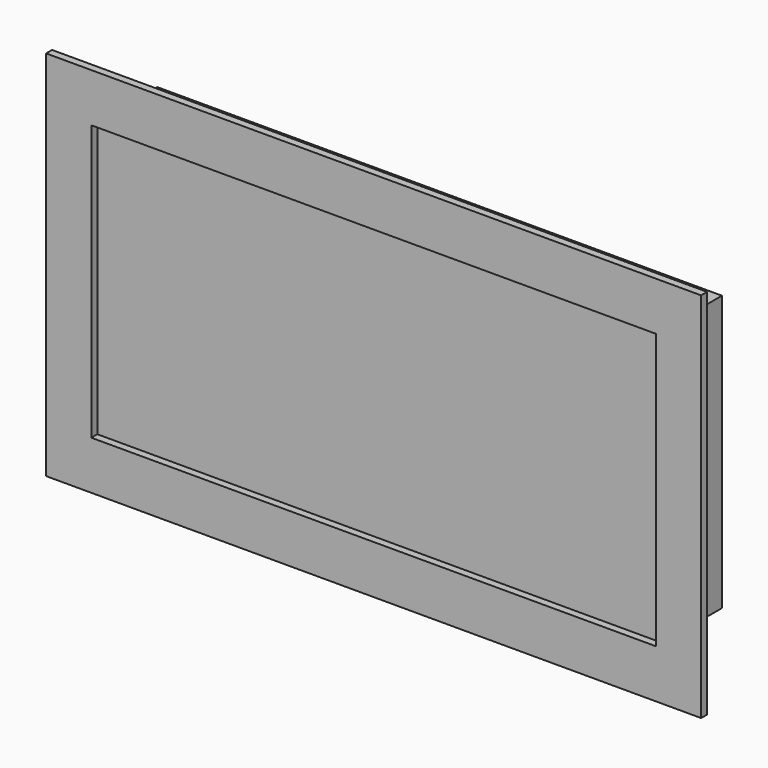
from build123d import *

# Parameters (mm, degrees)
F3_W     = 191.1528706551
F3_H     = 93.1293070316
F0_DEPTH = 25.4
F3_W_2   = 221.7658758163
F3_H_2   = 125.9914338589
F1_DEPTH = 2.54


# Not quite as in the source:
# - a feature of the source that left no trace in its solid (it failed there, or was rolled back) is left out


with BuildPart() as f0:
    # F3 (on Front) → F0 (new body)
    with BuildSketch(Plane.XZ):
        Rectangle(F3_W, F3_H)
    extrude(amount=-F0_DEPTH)


with BuildPart() as f1:
    # F3 (on Front) → F1 (new body)
    with BuildSketch(Plane.XZ):
        Rectangle(F3_W_2, F3_H_2)
        Rectangle(F3_W, F3_H, mode=Mode.SUBTRACT)
    extrude(amount=F1_DEPTH)


solid = Compound([f0.part, f1.part])
